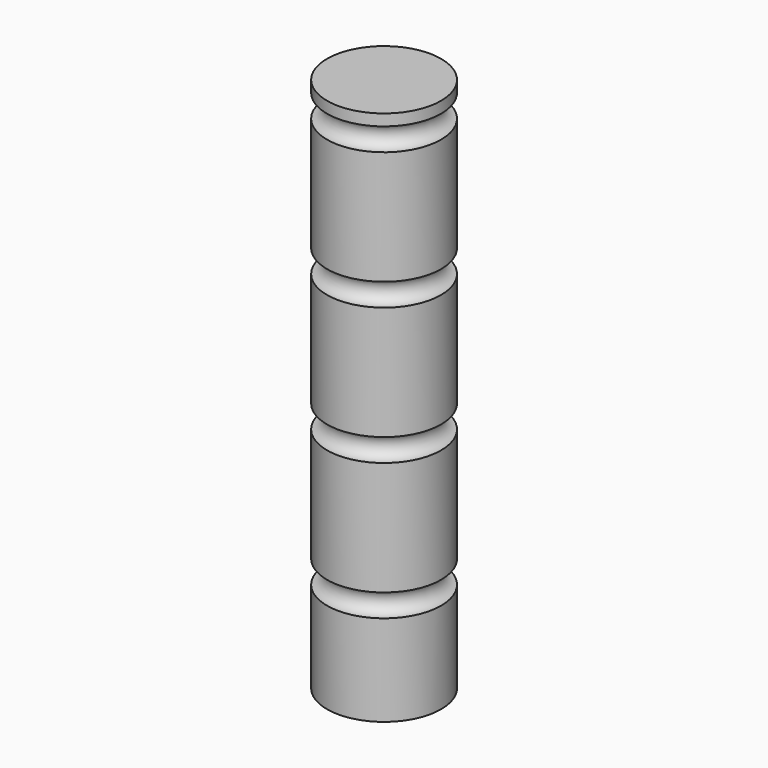
from build123d import *

# Parameters (mm, degrees)
F0_R      = 3.96875
F1_DEPTH  = 101.6
F2_W      = 3.96875
F2_H      = 64.29375
F4_W      = 7.9375
F4_H      = 7.9375
F5_DEPTH  = 7.9375
F7_DEPTH  = 7.9375
F8_R      = 3.96874
F12_W     = 1.56845
F12_H     = 1.6891
F12_W_2   = 1.6891
F12_H_2   = 1.56845
F13_DEPTH = 15.875
F14_W     = 27.7553014457
F14_H     = 25.7534027915
F15_DEPTH = 25.4


# Not quite as in the source:
# - a fillet or chamfer is up to 0.001 mm smaller than in the source, because OpenCascade refuses the exact size


with BuildPart() as f1:
    # F0 (on Top) → F1 (new body)
    with BuildSketch(Plane.XY):
        Circle(F0_R)
    extrude(amount=F1_DEPTH)

    # F2 (on Front) → F3 (revolve, cut)
    with BuildSketch(Plane.XZ):
        with BuildLine():
            Line((3.96875, 6.35), (3.96875, 7.9375))
            ThreePointArc((3.96875, 7.9375), (3.175, 7.14375), (3.96875, 6.35))
        make_face()
        with BuildLine():
            ThreePointArc((3.96875, 17.4625), (3.175, 16.66875), (3.96875, 15.875))
            Line((3.96875, 15.875), (3.96875, 17.4625))
        make_face()
        with BuildLine():
            ThreePointArc((3.96875, 26.9875), (3.175, 26.19375), (3.96875, 25.4))
            Line((3.96875, 25.4), (3.96875, 26.9875))
        make_face()
        with BuildLine():
            ThreePointArc((3.96875, 36.5125), (3.175, 35.71875), (3.96875, 34.925))
            Line((3.96875, 34.925), (3.96875, 36.5125))
        make_face()
        with Locations((1.984375, 69.453125)):
            Rectangle(F2_W, F2_H)
    revolve(axis=Axis((0, 0, 101.6), (0, 0, 1)), mode=Mode.SUBTRACT)

    # F4 (on face) → F5 (join)
    with BuildSketch(Plane(origin=(0, 0, 0), x_dir=(1, 0, 0), z_dir=(0, 0, -1))):
        Rectangle(F4_W, F4_H)
    extrude(amount=F5_DEPTH)

    # F6 (on face) → F7 (join, through all)
    with BuildSketch(Plane(origin=(0, 3.96875, 0), x_dir=(-1, 0, 0), z_dir=(0, 1, 0))):
        Polygon((3.96875, -7.9375), (3.96875, -17.4625), (7.9375, -17.4625), (7.9375, -3.96875), (3.96875, 0), (3.96875, -3.96875), align=None)
        Polygon((-7.9375, -17.4625), (-3.96875, -17.4625), (-3.96875, -7.9375), (-3.96875, -3.96875), (-3.96875, 0), (-7.9375, -3.96875), align=None)
    extrude(amount=-F7_DEPTH)

    # F8 (radius 3.96875 in the source; OpenCascade refuses exactly that, so slightly less here)
    f8_edges = [f1.edges().sort_by_distance(p)[0] for p in [
        (-5.953125, -3.96875, -17.4625),
        (-5.953125, 3.96875, -17.4625),
        (5.953125, 3.96875, -17.4625),
        (5.953125, -3.96875, -17.4625),
    ]]
    fillet(f8_edges, radius=F8_R)

    # F10 (on offset) → F11 (revolve, cut)
    with BuildSketch(Plane(origin=(0, 0, 0), x_dir=(-1, 0, 0), z_dir=(0, 1, 0))):
        Polygon((-11.90625, -7.9375), (-3.96875, 0), (-11.90625, 0), align=None)
    revolve(axis=Axis((0, 0, 7.9375), (0, 0, 1)), mode=Mode.SUBTRACT)

    # F12 (on face) → F13 (cut, through all)
    with BuildSketch(Plane(origin=(-7.9375, 0, 0), x_dir=(0, -1, 0), z_dir=(-1, 0, 0))):
        with Locations((1.628775, -13.49375)):
            Rectangle(F12_W, F12_H)
        with Locations((0, -13.49375)):
            Rectangle(F12_W_2, F12_H)
        with Locations((0, -11.864975)):
            Rectangle(F12_W_2, F12_H_2)
        with Locations((-1.628775, -13.49375)):
            Rectangle(F12_W, F12_H)
        with Locations((0, -15.122525)):
            Rectangle(F12_W_2, F12_H_2)
    extrude(amount=-F13_DEPTH, mode=Mode.SUBTRACT)

    # F14 (on face) → F15 (cut)
    with BuildSketch(Plane.YZ.offset(7.9375)):
        with Locations((0.0419458374, -12.8767013957)):
            Rectangle(F14_W, F14_H)
    extrude(amount=-F15_DEPTH, mode=Mode.SUBTRACT)


solid = f1.part
